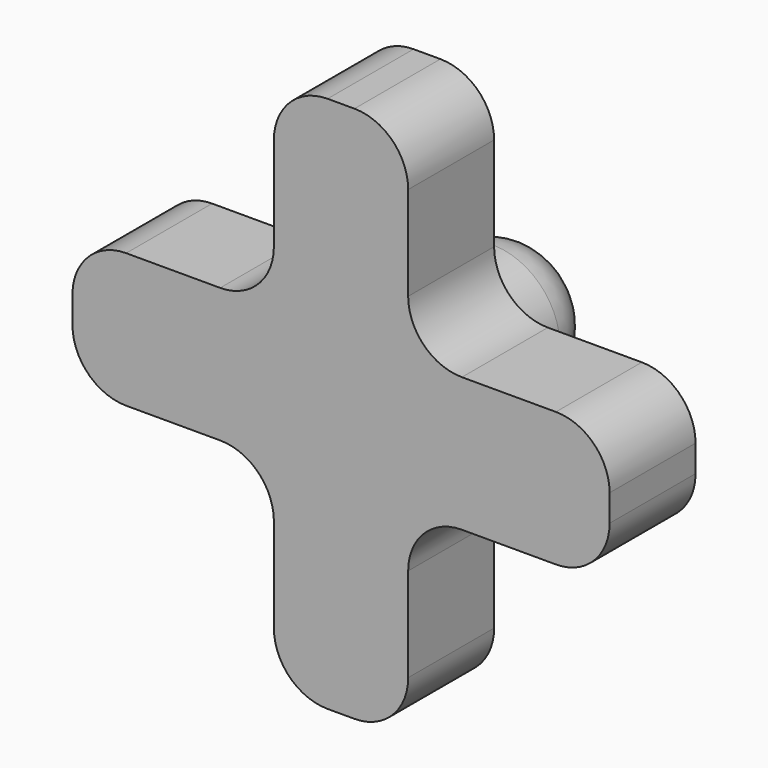
from build123d import *

# Parameters (mm, degrees)
F0_W     = 19.05
F0_H     = 12.7
F0_W_2   = 12.7
F0_H_2   = 19.05
F1_DEPTH = 10.16
F2_R     = 5.08
F3_R     = 6.35
F3_R_2   = 2.54
F4_DEPTH = 12.7
F5_DEPTH = 2.54


# Not quite as in the source:
# - a fillet or chamfer that OpenCascade refuses, or shapes differently, is made with other operations: its cross-section is extruded or revolved along the edge and cut away or added


with BuildPart() as f1:
    # F0 (on Front) → F1 (new body)
    with BuildSketch(Plane.XZ):
        with Locations((9.525, -6.35)):
            Rectangle(F0_W, F0_H)
        with Locations((25.4, 9.525)):
            Rectangle(F0_W_2, F0_H_2)
        with Locations((25.4, -6.35)):
            Rectangle(F0_W_2, F0_H)
        with Locations((41.275, -6.35)):
            Rectangle(F0_W, F0_H)
        with Locations((25.4, -22.225)):
            Rectangle(F0_W_2, F0_H_2)
    extrude(amount=F1_DEPTH)

    # F2
    f2_edges = [f1.edges().sort_by_distance(p)[0] for p in [
        (19.05, -5.08, -12.7),
        (19.05, -5.08, 0),
        (31.75, -5.08, 0),
        (31.75, -5.08, -12.7),
        (0, -5.08, 0),
        (0, -5.08, -12.7),
        (19.05, -5.08, -31.75),
        (31.75, -5.08, -31.75),
        (50.8, -5.08, -12.7),
        (50.8, -5.08, 0),
        (31.75, -5.08, 19.05),
        (19.05, -5.08, 19.05),
    ]]
    fillet(f2_edges, radius=F2_R)

    # F3 (on face) → F4 (join)
    with BuildSketch(Plane(origin=(0, 0, 0), x_dir=(-1, 0, 0), z_dir=(0, 1, 0))):
        with Locations((-25.4, -6.35)):
            Circle(F3_R)
        with Locations((-25.4, -6.35)):
            Circle(F3_R_2, mode=Mode.SUBTRACT)
    extrude(amount=F4_DEPTH)

    # F5 (cut): a face of the model
    f5_faces = [f1.faces().sort_by_distance(p)[0] for p in [
        (25.4, 0, -6.35),
    ]]
    extrude(f5_faces, amount=-F5_DEPTH, mode=Mode.SUBTRACT)

    # F6: fillet of radius 5.08 on 1 edges, made by hand

    # F6_s1 → F6_t2 (revolve, cut)
    with BuildSketch(Plane.XY.offset(-6.35)):
        with BuildLine():
            ThreePointArc((19.05, 7.7813111503), (20.1139073716, 10.8921631237), (22.86, 12.7))
            Line((22.86, 12.7), (19.05, 12.7))
            Line((19.05, 12.7), (19.05, 7.7813111503))
        make_face()
    revolve(axis=Axis((25.4, 12.7, -6.35), (0, 1, 0)), mode=Mode.SUBTRACT)


solid = f1.part
